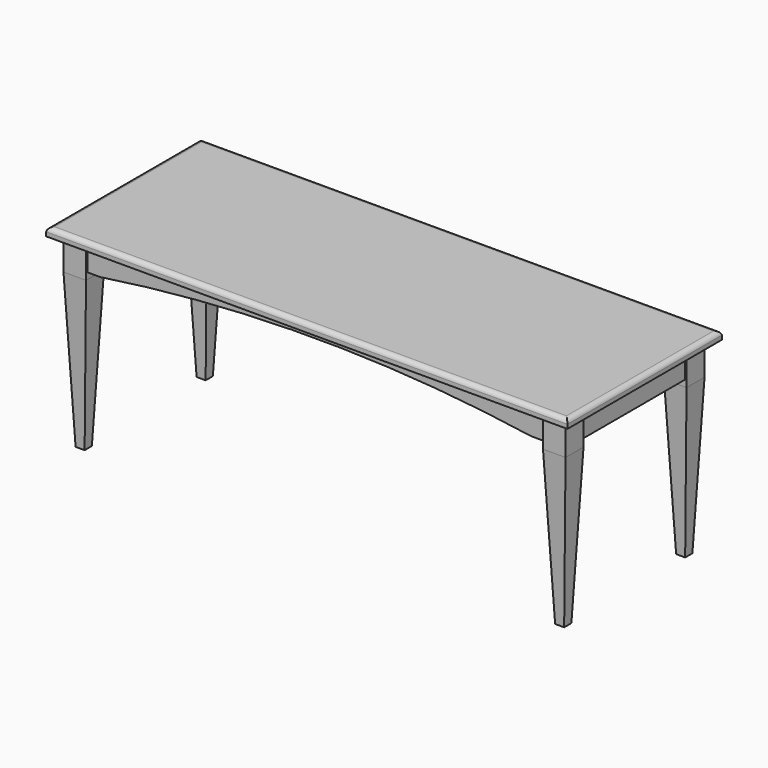
from build123d import *

# Parameters (mm, degrees)
F0_W           = 2057.4
F0_H           = 762
F1_DEPTH       = 15.875
F2_W           = 2057.4
F2_H           = 762
F3_DEPTH       = 15.875
F4_T1_DEPTH    = 2151.3177665567
F4_T3_DEPTH    = 855.9177665567
F6_W           = 88.9
F6_H           = 88.9
F7_DEPTH       = 127
F9_W           = 1968.5
F9_H           = 673.1
F10_DEPTH      = 101.6
F11_T          = -25.4
F12_W          = 88.9
F12_H          = 88.9
F13_DEPTH      = 609.6
F13_TAPER      = 2.5
F16_W          = 1701.8
F16_H          = 245.2263149261
F17_DEPTH      = 914.4
F17_DEPTH_BACK = 914.4


# Not quite as in the source:
# - a fillet or chamfer that OpenCascade refuses, or shapes differently, is made with other operations: its cross-section is extruded or revolved along the edge and cut away or added


with BuildPart() as f1:
    # F0 (on Top) → F1 (new body)
    with BuildSketch(Plane.XY):
        Rectangle(F0_W, F0_H)
    extrude(amount=F1_DEPTH)

    # F6 (on face) → F7 (join)
    with BuildSketch(Plane(origin=(0, 0, 0), x_dir=(1, 0, 0), z_dir=(0, 0, -1))):
        with Locations((-946.15, 298.45)):
            Rectangle(F6_W, F6_H)
        with Locations((-946.15, -298.45)):
            Rectangle(F6_W, F6_H)
    extrude(amount=F7_DEPTH)

    # F8: F1 across plane


with BuildPart() as f3:
    # F2 (on face) → F3 (new body)
    with BuildSketch(Plane.XY.offset(15.875)):
        Rectangle(F2_W, F2_H)
    extrude(amount=F3_DEPTH)

    # F4: fillet of radius 19.05 on 4 edges, made by hand

    # F4_s2 → F4_t1 (cut)
    with BuildSketch(Plane.YZ.offset(-1075.6588832784)):
        with BuildLine():
            ThreePointArc((-381, 15.875), (-374.5131688129, 27.2496778315), (-362.2164466887, 31.75))
            Line((-362.2164466887, 31.75), (-381, 31.75))
            Line((-381, 31.75), (-381, 15.875))
        make_face()
        with BuildLine():
            ThreePointArc((381, 15.875), (374.5131688129, 27.2496778315), (362.2164466887, 31.75))
            Line((362.2164466887, 31.75), (381, 31.75))
            Line((381, 31.75), (381, 15.875))
        make_face()
    extrude(amount=F4_T1_DEPTH, mode=Mode.SUBTRACT)

    # F4_s4 → F4_t3 (cut)
    with BuildSketch(Plane.XZ.offset(-427.9588832784)):
        with BuildLine():
            ThreePointArc((-1028.7, 15.875), (-1022.2131688129, 27.2496778315), (-1009.9164466887, 31.75))
            Line((-1009.9164466887, 31.75), (-1028.7, 31.75))
            Line((-1028.7, 31.75), (-1028.7, 15.875))
        make_face()
        with BuildLine():
            ThreePointArc((1028.7, 15.875), (1022.2131688129, 27.2496778315), (1009.9164466887, 31.75))
            Line((1009.9164466887, 31.75), (1028.7, 31.75))
            Line((1028.7, 31.75), (1028.7, 15.875))
        make_face()
    extrude(amount=F4_T3_DEPTH, mode=Mode.SUBTRACT)


with BuildPart() as f1_1:
    add(f1.part)
    add(f1.part.mirror(Plane.YZ))

    # F12 (on face) → F13 (join)
    with BuildSketch(Plane(origin=(0, 0, -127), x_dir=(1, 0, 0), z_dir=(0, 0, -1))):
        with Locations((-946.15, 298.45)):
            Rectangle(F12_W, F12_H)
    extrude(amount=F13_DEPTH, taper=F13_TAPER)


with BuildPart() as f10:
    # F9 (on face) → F10 (new body)
    with BuildSketch(Plane(origin=(0, 0, 0), x_dir=(1, 0, 0), z_dir=(0, 0, -1))):
        Rectangle(F9_W, F9_H)
    extrude(amount=F10_DEPTH)

    # F11
    f11_openings = [f10.faces().sort_by_distance(p)[0] for p in [
        (0, 0, -101.6),
    ]]
    offset(amount=F11_T, openings=f11_openings)

    # F16 (on Front) → F17 (cut, two sides)
    with BuildSketch(Plane.XZ) as f17_sk:
        with BuildLine():
            Line((-850.9, -101.6), (850.9, -101.6))
            ThreePointArc((850.9, -101.6), (0, -38.1), (-850.9, -101.6))
        make_face()
        with Locations((0, -224.2131574631)):
            Rectangle(F16_W, F16_H)
    extrude(amount=F17_DEPTH, mode=Mode.SUBTRACT)
    extrude(f17_sk.sketch, amount=-F17_DEPTH_BACK, mode=Mode.SUBTRACT)


with BuildPart() as f14_1:
    # F14: instance of F1
    add(f1_1.part.mirror(Plane.XZ))


with BuildPart() as f1_2:
    add(f1_1.part)

    add(f14_1.part)  # F15 merges F14_1
    # F15: F1, F14_1 across plane
    add(f1_1.part.mirror(Plane.YZ))
    add(f14_1.part.mirror(Plane.YZ))


solid = Compound([f3.part, f10.part, f1_2.part])
